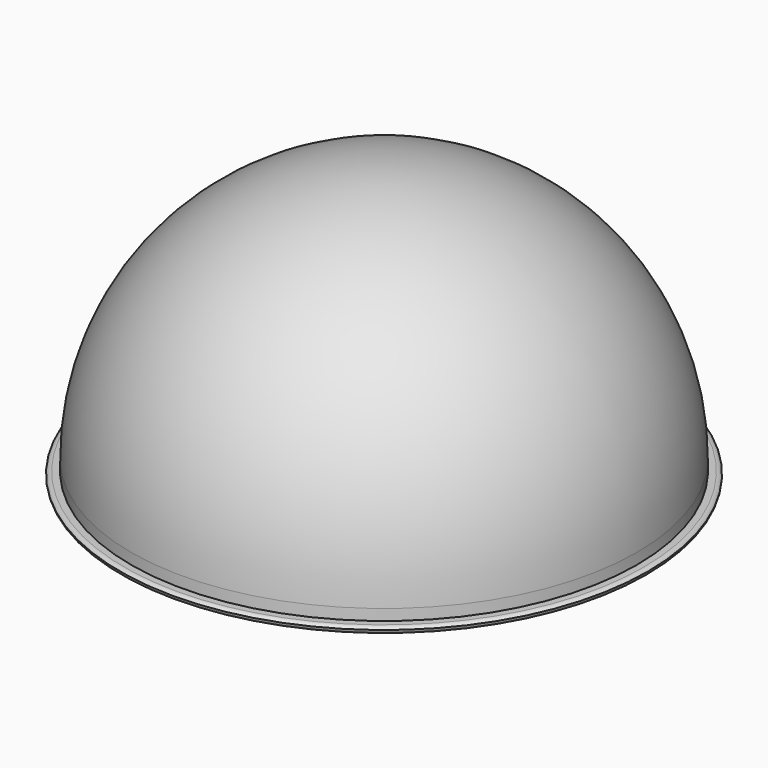
from build123d import *

# Parameters (mm, degrees)
F0_R      = 115
F1_DEPTH  = 120
F2_R      = 115
F3_R      = 120
F4_DEPTH  = 3
F5_R      = 2
F7_R      = 12.5
F8_DEPTH  = 25
F9_R      = 3
F10_DEPTH = 2
F11_R     = 1
F12_R     = 2


# Not quite as in the source:
# - a fillet or chamfer that OpenCascade refuses, or shapes differently, is made with other operations: its cross-section is extruded or revolved along the edge and cut away or added


with BuildPart() as f1:
    # F0 (on Top) → F1 (new body)
    with BuildSketch(Plane.XY):
        Circle(F0_R)
    extrude(amount=F1_DEPTH)

    # F2
    f2_edges = [f1.edges().sort_by_distance(p)[0] for p in [
        (-115, 0, 120),
    ]]
    fillet(f2_edges, radius=F2_R)

    # F3 (on face) → F4 (join)
    with BuildSketch(Plane(origin=(0, 0, 0), x_dir=(1, 0, 0), z_dir=(0, 0, -1))):
        Circle(F3_R)
        with BuildLine():
            Line((-2.8004212099, -2.5565289863), (-2.8004212099, -109.964347136))
            ThreePointArc((-2.8004212099, -109.964347136), (-77.8854638737, -77.6778895), (-109.9714289755, -2.5069521507))
            Line((-109.9714289755, -2.5069521507), (-2.8004212099, -2.5565289863))
        make_face(mode=Mode.SUBTRACT)
        with BuildLine():
            ThreePointArc((109.9690624994, -2.6086956522), (77.6369255508, -77.9262971725), (2.199560132, -109.9780065978))
            Line((2.199560132, -109.9780065978), (2.199560132, -2.5588419556))
            Line((2.199560132, -2.5588419556), (109.9690624994, -2.6086956522))
        make_face(mode=Mode.SUBTRACT)
        with BuildLine():
            Line((-2.8004212099, 2.6010809458), (-109.964347136, 2.8004212099))
            ThreePointArc((-109.964347136, 2.8004212099), (-77.7817459305, 77.7817459305), (-2.8004212099, 109.964347136))
            Line((-2.8004212099, 109.964347136), (-2.8004212099, 2.6010809458))
        make_face(mode=Mode.SUBTRACT)
        with BuildLine():
            ThreePointArc((2.199560132, 109.9780065978), (77.7139097925, 77.8495229578), (109.9740044898, 2.3913043478))
            Line((109.9740044898, 2.3913043478), (2.199560132, 2.5917802638))
            Line((2.199560132, 2.5917802638), (2.199560132, 109.9780065978))
        make_face(mode=Mode.SUBTRACT)
    extrude(amount=F4_DEPTH)

    # F5
    f5_edges = [f1.edges().sort_by_distance(p)[0] for p in [
        (-56.382384, -2.700751, -3),
        (-56.385925, 2.531741, -3),
        (-2.800421, 56.260438, -3),
        (2.19956, 56.268424, -3),
        (56.086782, -2.491542, -3),
        (56.084311, 2.583769, -3),
        (2.19956, -56.284893, -3),
        (-2.800421, -56.282714, -3),
        (-77.781746, -77.781746, -3),
        (-77.885464, 77.67789, -3),
        (-120, 0, -3),
        (77.71391, -77.849523, -3),
        (77.636926, 77.926297, -3),
    ]]
    fillet(f5_edges, radius=F5_R)

    # F6: fillet of radius 2.5 on 1 edges, made by hand

    # F6_s1 → F6_t2 (revolve, cut)
    with BuildSketch(Plane.XZ):
        with BuildLine():
            ThreePointArc((120, -1), (119.1180339887, -0.2639320225), (118, 0))
            Line((118, 0), (120, 0))
            Line((120, 0), (120, -1))
        make_face()
    revolve(axis=Axis((0, 0, 0), (0, 0, -1)), mode=Mode.SUBTRACT)

    # F7 (on face) → F8 (join)
    with BuildSketch(Plane(origin=(0, 0, 0), x_dir=(1, 0, 0), z_dir=(0, 0, -1))):
        Circle(F7_R)
    extrude(amount=F8_DEPTH)

    # F9 (on face) → F10 (join)
    with BuildSketch(Plane(origin=(0, 0, -25), x_dir=(1, 0, 0), z_dir=(0, 0, -1))):
        Circle(F9_R)
    extrude(amount=F10_DEPTH)

    # F11
    f11_edges = [f1.edges().sort_by_distance(p)[0] for p in [
        (-3, 0, -27),
    ]]
    fillet(f11_edges, radius=F11_R)

    # F12
    f12_edges = [f1.edges().sort_by_distance(p)[0] for p in [
        (-12.5, 0, -25),
    ]]
    fillet(f12_edges, radius=F12_R)


solid = f1.part
